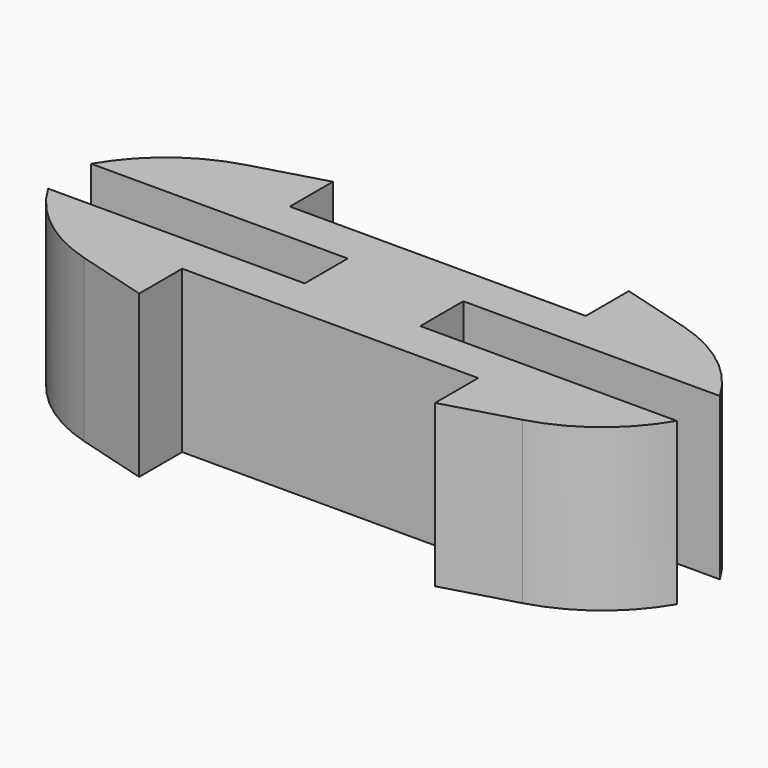
from build123d import *

# Parameters (mm, degrees)
F1_DEPTH    = 6
F2_T1_DEPTH = 28.6290423826
F3_W        = 12.6199351555
F3_H        = 2
F3_W_2      = 15.3329153147
F4_DEPTH    = 6


# Not quite as in the source:
# - a fillet or chamfer that OpenCascade refuses, or shapes differently, is made with other operations: its cross-section is extruded or revolved along the edge and cut away or added


with BuildPart() as f1:
    # F0 (on Top) → F1 (new body)
    with BuildSketch(Plane.XY):
        Polygon((0, 7), (-7, 5), (0, 5), align=None)
        Polygon((0, 5), (-7, 5), (-7, 0), (0, 0), (11, 0), (18, 0), (18, 5), (11, 5), align=None)
        Polygon((0, 0), (-7, 0), (0, -2), align=None)
        Polygon((11, 7), (11, 5), (18, 5), align=None)
        Polygon((18, 0), (11, 0), (11, -2), align=None)
    extrude(amount=F1_DEPTH)

    # F2: fillet of radius 6 on 4 edges, made by hand

    # F2_s2 → F2_t1 (cut)
    with BuildSketch(Plane.XY.offset(-11.3145211913)):
        with BuildLine():
            ThreePointArc((-2.6483267674, 6.2433352093), (-5.7900918887, 4.0873646023), (-7, 0.4741915235))
            Line((-7, 0.4741915235), (-7, 5))
            Line((-7, 5), (-2.6483267674, 6.2433352093))
        make_face()
        with BuildLine():
            ThreePointArc((-7, 4.5258084765), (-5.7900918887, 0.9126353977), (-2.6483267674, -1.2433352093))
            Line((-2.6483267674, -1.2433352093), (-7, 0))
            Line((-7, 0), (-7, 4.5258084765))
        make_face()
        with BuildLine():
            ThreePointArc((18, 0.4741915235), (16.7900918887, 4.0873646023), (13.6483267674, 6.2433352093))
            Line((13.6483267674, 6.2433352093), (18, 5))
            Line((18, 5), (18, 0.4741915235))
        make_face()
        with BuildLine():
            ThreePointArc((13.6483267674, -1.2433352093), (16.7900918887, 0.9126353977), (18, 4.5258084765))
            Line((18, 4.5258084765), (18, 0))
            Line((18, 0), (13.6483267674, -1.2433352093))
        make_face()
    extrude(amount=F2_T1_DEPTH, mode=Mode.SUBTRACT)

    # F3 (on face) → F4 (cut)
    with BuildSketch(Plane.XY.offset(6)):
        with Locations((-2.9576308128, 2.5)):
            Rectangle(F3_W, F3_H)
        with Locations((15.3141208924, 2.5)):
            Rectangle(F3_W_2, F3_H)
    extrude(amount=-F4_DEPTH, mode=Mode.SUBTRACT)


solid = f1.part
